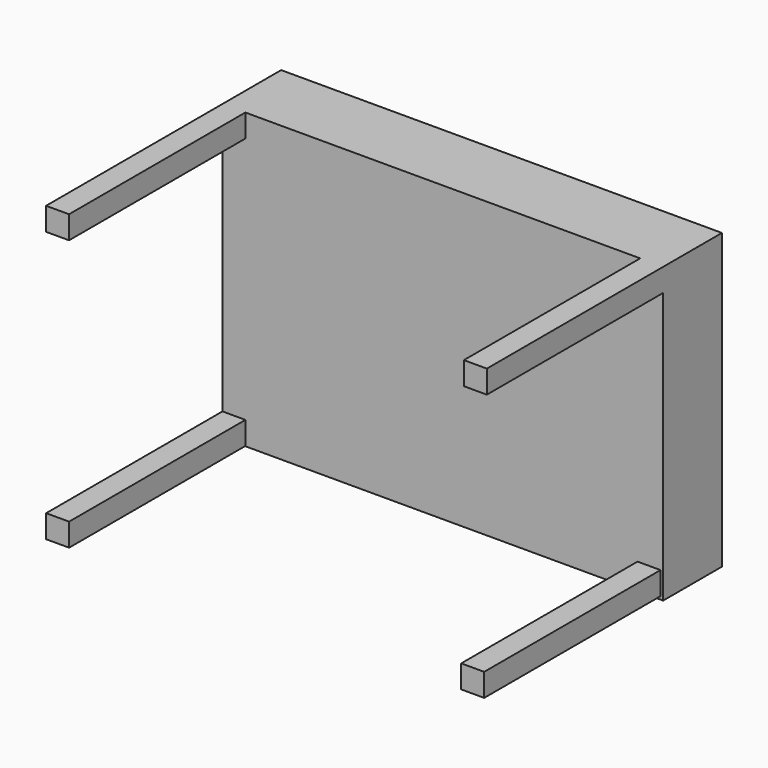
from build123d import *

# Parameters (mm, degrees)
F0_W      = 152.4
F0_H      = 101.6
F1_DEPTH  = 25.4
F2_W      = 7.9375
F2_H      = 7.9375
F3_DEPTH  = 76.2
F4_W      = 7.9375
F4_H      = 7.9375
F7_DEPTH  = 76.2
F5_W      = 7.9375
F5_H      = 7.9375
F8_DEPTH  = 76.2
F6_W      = 7.9375
F6_H      = 7.9375
F9_DEPTH  = 76.2
F10_W     = 136.525
F10_H     = 85.725
F11_DEPTH = 12.7


# Not quite as in the source:
# - a length typed as a fraction of an inch, garbled in the dataset ("3 / 203.2 mm" for 3/8 in), is restored


with BuildPart() as f1:
    # F0 (on Front) → F1 (new body)
    with BuildSketch(Plane.XZ):
        with Locations((-82.3848899454, 39.5816343878)):
            Rectangle(F0_W, F0_H)
    extrude(amount=F1_DEPTH)

    # F2 (on face) → F3 (join)
    with BuildSketch(Plane.XZ.offset(25.4)):
        with Locations((-154.6161399454, 86.4128843878)):
            Rectangle(F2_W, F2_H)
    extrude(amount=F3_DEPTH)

    # F4 (on face) → F7 (join)
    with BuildSketch(Plane.XZ.offset(25.4)):
        with Locations((-10.1536399454, 86.4128843878)):
            Rectangle(F4_W, F4_H)
    extrude(amount=F7_DEPTH)

    # F5 (on face) → F8 (join)
    with BuildSketch(Plane.XZ.offset(25.4)):
        with Locations((-154.5934006572, -7.1469780084)):
            Rectangle(F5_W, F5_H)
    extrude(amount=F8_DEPTH)

    # F6 (on face) → F9 (join)
    with BuildSketch(Plane.XZ.offset(25.4)):
        with Locations((-11.0744582489, -6.1915257747)):
            Rectangle(F6_W, F6_H)
    extrude(amount=F9_DEPTH)

    # F10 (on face) → F11 (cut)
    with BuildSketch(Plane(origin=(0, 0, 0), x_dir=(-1, 0, 0), z_dir=(0, 1, 0))):
        with Locations((82.3848899454, 39.5816343878)):
            Rectangle(F10_W, F10_H)
    extrude(amount=-F11_DEPTH, mode=Mode.SUBTRACT)


solid = f1.part
